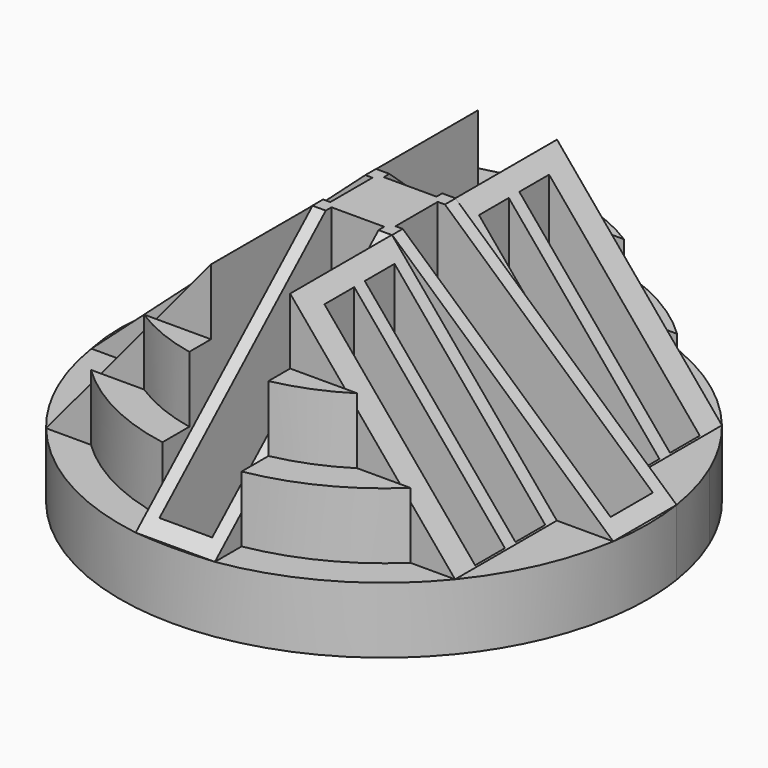
from build123d import *
from build123d import SkipClean  # not in build123d's __all__

# Parameters (mm, degrees)
F2_DEPTH  = 12.7
F3_DEPTH  = 25.4
F4_DEPTH  = 38.1
F5_DEPTH  = 50.8
F6_DEPTH  = 50.8
F7_DEPTH  = 50.8
F11_DEPTH = 15.24
F12_DEPTH = 15.24
F13_DEPTH = 15.24
F15_DEPTH = 15.24
F16_W     = 41.402
F16_H     = 10.16
F16_W_2   = 10.16
F16_H_2   = 41.402
F17_DEPTH = 44.45
F18_DEPTH = 50.8
F21_DEPTH = 24.4856
F19_W     = 29.0068
F19_H     = 7.1628
F22_DEPTH = 44.45
F24_DEPTH = 24.4856
F26_DEPTH = 24.4856
F28_DEPTH = 24.4856


# Not quite as in the source:
# - a feature names something its author has since deleted; it is built from what else it names


with BuildPart() as f2:
    # F1 (on Top) → F2 (new body)
    with BuildSketch(Plane.XY):
        with BuildLine():
            Line((-7.62, 43.7919867099), (-7.62, 50.2252486305))
            ThreePointArc((-7.62, 50.2252486305), (-25.1805025773, 44.1200894146), (-39.3683940318, 32.1056))
            Line((-39.3683940318, 32.1056), (-30.7413882029, 32.1056))
            ThreePointArc((-30.7413882029, 32.1056), (-20.0509833873, 39.670651182), (-7.62, 43.7919867099))
        make_face()
        with BuildLine():
            Line((-30.7413882029, 32.1056), (-39.3683940318, 32.1056))
            ThreePointArc((-39.3683940318, 32.1056), (-43.4950311771, 26.2454236564), (-46.7558464383, 19.8628))
            Line((-46.7558464383, 19.8628), (-39.7652068542, 19.8628))
            ThreePointArc((-39.7652068542, 19.8628), (-35.7808122406, 26.3730160468), (-30.7413882029, 32.1056))
        make_face()
        with BuildLine():
            Line((-39.7652068542, 19.8628), (-46.7558464383, 19.8628))
            ThreePointArc((-46.7558464383, 19.8628), (-48.8754001329, 13.850460709), (-50.2252486305, 7.62))
            Line((-50.2252486305, 7.62), (-43.7919867099, 7.62))
            ThreePointArc((-43.7919867099, 7.62), (-42.2246691762, 13.8881176896), (-39.7652068542, 19.8628))
        make_face()
        with BuildLine():
            Line((-43.7919867099, 7.62), (-50.2252486305, 7.62))
            ThreePointArc((-50.2252486305, 7.62), (-50.8, 0), (-50.2252486305, -7.62))
            Line((-50.2252486305, -7.62), (-43.7919867099, -7.62))
            ThreePointArc((-43.7919867099, -7.62), (-44.45, 0), (-43.7919867099, 7.62))
        make_face()
        with BuildLine():
            ThreePointArc((-50.2252486305, -7.62), (-48.8754001329, -13.850460709), (-46.7558464383, -19.8628))
            Line((-46.7558464383, -19.8628), (-39.7652068542, -19.8628))
            ThreePointArc((-39.7652068542, -19.8628), (-42.2246691762, -13.8881176896), (-43.7919867099, -7.62))
            Line((-43.7919867099, -7.62), (-50.2252486305, -7.62))
        make_face()
        with BuildLine():
            ThreePointArc((-46.7558464383, -19.8628), (-43.4950311771, -26.2454236564), (-39.3683940318, -32.1056))
            Line((-39.3683940318, -32.1056), (-30.7413882029, -32.1056))
            ThreePointArc((-30.7413882029, -32.1056), (-35.7808122406, -26.3730160468), (-39.7652068542, -19.8628))
            Line((-39.7652068542, -19.8628), (-46.7558464383, -19.8628))
        make_face()
        with BuildLine():
            ThreePointArc((-39.3683940318, -32.1056), (-25.1805025773, -44.1200894146), (-7.62, -50.2252486305))
            Line((-7.62, -50.2252486305), (-7.62, -43.7919867099))
            ThreePointArc((-7.62, -43.7919867099), (-20.0509833873, -39.670651182), (-30.7413882029, -32.1056))
            Line((-30.7413882029, -32.1056), (-39.3683940318, -32.1056))
        make_face()
        with BuildLine():
            Line((7.62, 43.7919867099), (7.62, 50.2252486305))
            ThreePointArc((7.62, 50.2252486305), (0, 50.8), (-7.62, 50.2252486305))
            Line((-7.62, 50.2252486305), (-7.62, 43.7919867099))
            ThreePointArc((-7.62, 43.7919867099), (0, 44.45), (7.62, 43.7919867099))
        make_face()
        with BuildLine():
            ThreePointArc((7.62, -50.2252486305), (25.1805025773, -44.1200894146), (39.3683940318, -32.1056))
            Line((39.3683940318, -32.1056), (30.7413882029, -32.1056))
            ThreePointArc((30.7413882029, -32.1056), (20.0509833873, -39.670651182), (7.62, -43.7919867099))
            Line((7.62, -43.7919867099), (7.62, -50.2252486305))
        make_face()
        with BuildLine():
            ThreePointArc((39.3683940318, -32.1056), (43.4950311771, -26.2454236564), (46.7558464383, -19.8628))
            Line((46.7558464383, -19.8628), (39.7652068542, -19.8628))
            ThreePointArc((39.7652068542, -19.8628), (35.7808122406, -26.3730160468), (30.7413882029, -32.1056))
            Line((30.7413882029, -32.1056), (39.3683940318, -32.1056))
        make_face()
        with BuildLine():
            ThreePointArc((46.7558464383, -19.8628), (48.8754001329, -13.850460709), (50.2252486305, -7.62))
            Line((50.2252486305, -7.62), (43.7919867099, -7.62))
            ThreePointArc((43.7919867099, -7.62), (42.2246691762, -13.8881176896), (39.7652068542, -19.8628))
            Line((39.7652068542, -19.8628), (46.7558464383, -19.8628))
        make_face()
        with BuildLine():
            ThreePointArc((50.2252486305, -7.62), (50.6561083702, -3.8208225272), (50.8, 0))
            ThreePointArc((50.8, 0), (50.6561083702, 3.8208225272), (50.2252486305, 7.62))
            Line((50.2252486305, 7.62), (43.7919867099, 7.62))
            ThreePointArc((43.7919867099, 7.62), (44.45, 0), (43.7919867099, -7.62))
            Line((43.7919867099, -7.62), (50.2252486305, -7.62))
        make_face()
        with BuildLine():
            Line((43.7919867099, 7.62), (50.2252486305, 7.62))
            ThreePointArc((50.2252486305, 7.62), (48.8754001329, 13.850460709), (46.7558464383, 19.8628))
            Line((46.7558464383, 19.8628), (39.7652068542, 19.8628))
            ThreePointArc((39.7652068542, 19.8628), (42.2246691762, 13.8881176896), (43.7919867099, 7.62))
        make_face()
        with BuildLine():
            Line((39.7652068542, 19.8628), (46.7558464383, 19.8628))
            ThreePointArc((46.7558464383, 19.8628), (43.4950311771, 26.2454236564), (39.3683940318, 32.1056))
            Line((39.3683940318, 32.1056), (30.7413882029, 32.1056))
            ThreePointArc((30.7413882029, 32.1056), (35.7808122406, 26.3730160468), (39.7652068542, 19.8628))
        make_face()
        with BuildLine():
            Line((30.7413882029, 32.1056), (39.3683940318, 32.1056))
            ThreePointArc((39.3683940318, 32.1056), (25.1805025773, 44.1200894146), (7.62, 50.2252486305))
            Line((7.62, 50.2252486305), (7.62, 43.7919867099))
            ThreePointArc((7.62, 43.7919867099), (20.0509833873, 39.670651182), (30.7413882029, 32.1056))
        make_face()
        with BuildLine():
            ThreePointArc((-7.62, -50.2252486305), (0, -50.8), (7.62, -50.2252486305))
            Line((7.62, -50.2252486305), (7.62, -43.7919867099))
            ThreePointArc((7.62, -43.7919867099), (0, -44.45), (-7.62, -43.7919867099))
            Line((-7.62, -43.7919867099), (-7.62, -50.2252486305))
        make_face()
    extrude(amount=F2_DEPTH)

    # F1 (on Top) → F3 (join)
    with BuildSketch(Plane.XY):
        with BuildLine():
            ThreePointArc((7.62, -43.7919867099), (20.0509833873, -39.670651182), (30.7413882029, -32.1056))
            Line((30.7413882029, -32.1056), (20.5143961315, -32.1056))
            ThreePointArc((20.5143961315, -32.1056), (14.3076984372, -35.3114679025), (7.62, -37.33022368))
            Line((7.62, -37.33022368), (7.62, -43.7919867099))
        make_face()
        with BuildLine():
            ThreePointArc((30.7413882029, -32.1056), (35.7808122406, -26.3730160468), (39.7652068542, -19.8628))
            Line((39.7652068542, -19.8628), (32.5127540538, -19.8628))
            ThreePointArc((32.5127540538, -19.8628), (27.2110492659, -26.667748271), (20.5143961315, -32.1056))
            Line((20.5143961315, -32.1056), (30.7413882029, -32.1056))
        make_face()
        with BuildLine():
            ThreePointArc((39.7652068542, -19.8628), (42.2246691762, -13.8881176896), (43.7919867099, -7.62))
            Line((43.7919867099, -7.62), (37.33022368, -7.62))
            ThreePointArc((37.33022368, -7.62), (35.4539408619, -13.9509167211), (32.5127540538, -19.8628))
            Line((32.5127540538, -19.8628), (39.7652068542, -19.8628))
        make_face()
        with BuildLine():
            ThreePointArc((43.7919867099, -7.62), (44.45, 0), (43.7919867099, 7.62))
            Line((43.7919867099, 7.62), (37.33022368, 7.62))
            ThreePointArc((37.33022368, 7.62), (38.1, 0), (37.33022368, -7.62))
            Line((37.33022368, -7.62), (43.7919867099, -7.62))
        make_face()
        with BuildLine():
            Line((37.33022368, 7.62), (43.7919867099, 7.62))
            ThreePointArc((43.7919867099, 7.62), (42.2246691762, 13.8881176896), (39.7652068542, 19.8628))
            Line((39.7652068542, 19.8628), (32.5127540538, 19.8628))
            ThreePointArc((32.5127540538, 19.8628), (35.4539408619, 13.9509167211), (37.33022368, 7.62))
        make_face()
        with BuildLine():
            Line((32.5127540538, 19.8628), (39.7652068542, 19.8628))
            ThreePointArc((39.7652068542, 19.8628), (35.7808122406, 26.3730160468), (30.7413882029, 32.1056))
            Line((30.7413882029, 32.1056), (20.5143961315, 32.1056))
            ThreePointArc((20.5143961315, 32.1056), (27.2110492659, 26.667748271), (32.5127540538, 19.8628))
        make_face()
        with BuildLine():
            Line((20.5143961315, 32.1056), (30.7413882029, 32.1056))
            ThreePointArc((30.7413882029, 32.1056), (20.0509833873, 39.670651182), (7.62, 43.7919867099))
            Line((7.62, 43.7919867099), (7.62, 37.33022368))
            ThreePointArc((7.62, 37.33022368), (14.3076984372, 35.3114679025), (20.5143961315, 32.1056))
        make_face()
        with BuildLine():
            Line((7.62, 37.33022368), (7.62, 43.7919867099))
            ThreePointArc((7.62, 43.7919867099), (0, 44.45), (-7.62, 43.7919867099))
            Line((-7.62, 43.7919867099), (-7.62, 37.33022368))
            ThreePointArc((-7.62, 37.33022368), (0, 38.1), (7.62, 37.33022368))
        make_face()
        with BuildLine():
            ThreePointArc((-7.62, -43.7919867099), (0, -44.45), (7.62, -43.7919867099))
            Line((7.62, -43.7919867099), (7.62, -37.33022368))
            ThreePointArc((7.62, -37.33022368), (0, -38.1), (-7.62, -37.33022368))
            Line((-7.62, -37.33022368), (-7.62, -43.7919867099))
        make_face()
        with BuildLine():
            Line((-37.33022368, 7.62), (-43.7919867099, 7.62))
            ThreePointArc((-43.7919867099, 7.62), (-44.45, 0), (-43.7919867099, -7.62))
            Line((-43.7919867099, -7.62), (-37.33022368, -7.62))
            ThreePointArc((-37.33022368, -7.62), (-38.1, 0), (-37.33022368, 7.62))
        make_face()
        with BuildLine():
            ThreePointArc((-43.7919867099, -7.62), (-42.2246691762, -13.8881176896), (-39.7652068542, -19.8628))
            Line((-39.7652068542, -19.8628), (-32.5127540538, -19.8628))
            ThreePointArc((-32.5127540538, -19.8628), (-35.4539408619, -13.9509167211), (-37.33022368, -7.62))
            Line((-37.33022368, -7.62), (-43.7919867099, -7.62))
        make_face()
        with BuildLine():
            ThreePointArc((-39.7652068542, -19.8628), (-35.7808122406, -26.3730160468), (-30.7413882029, -32.1056))
            Line((-30.7413882029, -32.1056), (-20.5143961315, -32.1056))
            ThreePointArc((-20.5143961315, -32.1056), (-27.2110492659, -26.667748271), (-32.5127540538, -19.8628))
            Line((-32.5127540538, -19.8628), (-39.7652068542, -19.8628))
        make_face()
        with BuildLine():
            ThreePointArc((-30.7413882029, -32.1056), (-20.0509833873, -39.670651182), (-7.62, -43.7919867099))
            Line((-7.62, -43.7919867099), (-7.62, -37.33022368))
            ThreePointArc((-7.62, -37.33022368), (-14.2009349705, -35.3545392554), (-20.32, -32.2289869527))
            ThreePointArc((-20.32, -32.2289869527), (-20.4172912734, -32.1674403249), (-20.5143961315, -32.1056))
            Line((-20.5143961315, -32.1056), (-30.7413882029, -32.1056))
        make_face()
        with BuildLine():
            Line((-32.5127540538, 19.8628), (-39.7652068542, 19.8628))
            ThreePointArc((-39.7652068542, 19.8628), (-42.2246691762, 13.8881176896), (-43.7919867099, 7.62))
            Line((-43.7919867099, 7.62), (-37.33022368, 7.62))
            ThreePointArc((-37.33022368, 7.62), (-35.4539408619, 13.9509167211), (-32.5127540538, 19.8628))
        make_face()
        with BuildLine():
            Line((-20.5143961315, 32.1056), (-30.7413882029, 32.1056))
            ThreePointArc((-30.7413882029, 32.1056), (-35.7808122406, 26.3730160468), (-39.7652068542, 19.8628))
            Line((-39.7652068542, 19.8628), (-32.5127540538, 19.8628))
            ThreePointArc((-32.5127540538, 19.8628), (-27.2110492659, 26.667748271), (-20.5143961315, 32.1056))
        make_face()
        with BuildLine():
            Line((-7.62, 37.33022368), (-7.62, 43.7919867099))
            ThreePointArc((-7.62, 43.7919867099), (-20.0509833873, 39.670651182), (-30.7413882029, 32.1056))
            Line((-30.7413882029, 32.1056), (-20.5143961315, 32.1056))
            ThreePointArc((-20.5143961315, 32.1056), (-14.3076984372, 35.3114679025), (-7.62, 37.33022368))
        make_face()
    extrude(amount=F3_DEPTH)

    # F1 (on Top) → F4 (join)
    with BuildSketch(Plane.XY):
        with BuildLine():
            ThreePointArc((-7.62, -37.33022368), (0, -38.1), (7.62, -37.33022368))
            Line((7.62, -37.33022368), (7.62, -32.1056))
            Line((7.62, -32.1056), (7.62, -30.8220391928))
            ThreePointArc((7.62, -30.8220391928), (0, -31.75), (-7.62, -30.8220391928))
            Line((-7.62, -30.8220391928), (-7.62, -32.1056))
            Line((-7.62, -32.1056), (-7.62, -37.33022368))
        make_face()
        with BuildLine():
            Line((-7.62, 32.1056), (-7.62, 37.33022368))
            ThreePointArc((-7.62, 37.33022368), (-14.3076984372, 35.3114679025), (-20.5143961315, 32.1056))
            Line((-20.5143961315, 32.1056), (-7.62, 32.1056))
        make_face()
        with BuildLine():
            ThreePointArc((-30.8220391928, 7.62), (-28.4618751136, 14.0706845966), (-24.769571578, 19.8628))
            Line((-24.769571578, 19.8628), (-32.5127540538, 19.8628))
            ThreePointArc((-32.5127540538, 19.8628), (-35.4539408619, 13.9509167211), (-37.33022368, 7.62))
            Line((-37.33022368, 7.62), (-30.8220391928, 7.62))
        make_face()
        with BuildLine():
            Line((-20.32, -32.1056), (-20.5143961315, -32.1056))
            ThreePointArc((-20.5143961315, -32.1056), (-20.4172912734, -32.1674403249), (-20.32, -32.2289869527))
            Line((-20.32, -32.2289869527), (-20.32, -32.1056))
        make_face()
        with BuildLine():
            ThreePointArc((7.62, -37.33022368), (14.3076984372, -35.3114679025), (20.5143961315, -32.1056))
            Line((20.5143961315, -32.1056), (7.62, -32.1056))
            Line((7.62, -32.1056), (7.62, -37.33022368))
        make_face()
        with BuildLine():
            ThreePointArc((32.5127540538, -19.8628), (35.4539408619, -13.9509167211), (37.33022368, -7.62))
            Line((37.33022368, -7.62), (30.8220391928, -7.62))
            ThreePointArc((30.8220391928, -7.62), (28.4618751136, -14.0706845966), (24.769571578, -19.8628))
            Line((24.769571578, -19.8628), (32.5127540538, -19.8628))
        make_face()
        with BuildLine():
            Line((7.62, 32.1056), (20.5143961315, 32.1056))
            ThreePointArc((20.5143961315, 32.1056), (14.3076984372, 35.3114679025), (7.62, 37.33022368))
            Line((7.62, 37.33022368), (7.62, 32.1056))
        make_face()
        with BuildLine():
            Line((7.62, 32.1056), (7.62, 37.33022368))
            ThreePointArc((7.62, 37.33022368), (0, 38.1), (-7.62, 37.33022368))
            Line((-7.62, 37.33022368), (-7.62, 32.1056))
            Line((-7.62, 32.1056), (-7.62, 30.8220391928))
            ThreePointArc((-7.62, 30.8220391928), (0, 31.75), (7.62, 30.8220391928))
            Line((7.62, 30.8220391928), (7.62, 32.1056))
        make_face()
        with BuildLine():
            ThreePointArc((-24.769571578, 19.8628), (-17.0967048776, 26.7537881865), (-7.62, 30.8220391928))
            Line((-7.62, 30.8220391928), (-7.62, 32.1056))
            Line((-7.62, 32.1056), (-20.5143961315, 32.1056))
            ThreePointArc((-20.5143961315, 32.1056), (-27.2110492659, 26.667748271), (-32.5127540538, 19.8628))
            Line((-32.5127540538, 19.8628), (-24.769571578, 19.8628))
        make_face()
        with BuildLine():
            Line((24.769571578, 19.8628), (32.5127540538, 19.8628))
            ThreePointArc((32.5127540538, 19.8628), (27.2110492659, 26.667748271), (20.5143961315, 32.1056))
            Line((20.5143961315, 32.1056), (7.62, 32.1056))
            Line((7.62, 32.1056), (7.62, 30.8220391928))
            ThreePointArc((7.62, 30.8220391928), (17.0967048776, 26.7537881865), (24.769571578, 19.8628))
        make_face()
        with BuildLine():
            ThreePointArc((-30.8220391928, -7.62), (-31.75, 0), (-30.8220391928, 7.62))
            Line((-30.8220391928, 7.62), (-37.33022368, 7.62))
            ThreePointArc((-37.33022368, 7.62), (-38.1, 0), (-37.33022368, -7.62))
            Line((-37.33022368, -7.62), (-30.8220391928, -7.62))
        make_face()
        with BuildLine():
            Line((-32.5127540538, -19.8628), (-24.769571578, -19.8628))
            ThreePointArc((-24.769571578, -19.8628), (-28.4618751136, -14.0706845966), (-30.8220391928, -7.62))
            Line((-30.8220391928, -7.62), (-37.33022368, -7.62))
            ThreePointArc((-37.33022368, -7.62), (-35.4539408619, -13.9509167211), (-32.5127540538, -19.8628))
        make_face()
        with BuildLine():
            Line((-7.62, -32.1056), (-7.62, -30.8220391928))
            ThreePointArc((-7.62, -30.8220391928), (-17.0967048776, -26.7537881865), (-24.769571578, -19.8628))
            Line((-24.769571578, -19.8628), (-32.5127540538, -19.8628))
            ThreePointArc((-32.5127540538, -19.8628), (-27.2110492659, -26.667748271), (-20.5143961315, -32.1056))
            Line((-20.5143961315, -32.1056), (-20.32, -32.1056))
            Line((-20.32, -32.1056), (-7.62, -32.1056))
        make_face()
        with BuildLine():
            ThreePointArc((37.33022368, -7.62), (38.1, 0), (37.33022368, 7.62))
            Line((37.33022368, 7.62), (30.8220391928, 7.62))
            ThreePointArc((30.8220391928, 7.62), (31.5171559977, 3.8381477062), (31.75, 0))
            ThreePointArc((31.75, 0), (31.5171559977, -3.8381477062), (30.8220391928, -7.62))
            Line((30.8220391928, -7.62), (37.33022368, -7.62))
        make_face()
        with BuildLine():
            Line((30.8220391928, 7.62), (37.33022368, 7.62))
            ThreePointArc((37.33022368, 7.62), (35.4539408619, 13.9509167211), (32.5127540538, 19.8628))
            Line((32.5127540538, 19.8628), (24.769571578, 19.8628))
            ThreePointArc((24.769571578, 19.8628), (28.4618751136, 14.0706845966), (30.8220391928, 7.62))
        make_face()
        with BuildLine():
            ThreePointArc((-20.32, -32.2289869527), (-14.2009349705, -35.3545392554), (-7.62, -37.33022368))
            Line((-7.62, -37.33022368), (-7.62, -32.1056))
            Line((-7.62, -32.1056), (-20.32, -32.1056))
            Line((-20.32, -32.1056), (-20.32, -32.2289869527))
        make_face()
        with BuildLine():
            ThreePointArc((20.5143961315, -32.1056), (27.2110492659, -26.667748271), (32.5127540538, -19.8628))
            Line((32.5127540538, -19.8628), (24.769571578, -19.8628))
            ThreePointArc((24.769571578, -19.8628), (17.0967048776, -26.7537881865), (7.62, -30.8220391928))
            Line((7.62, -30.8220391928), (7.62, -32.1056))
            Line((7.62, -32.1056), (20.5143961315, -32.1056))
        make_face()
    extrude(amount=F4_DEPTH)

    # F1 (on Top) → F5 (join)
    with BuildSketch(Plane.XY):
        with BuildLine():
            Line((7.62, 24.230055716), (7.62, 30.8220391928))
            ThreePointArc((7.62, 30.8220391928), (0, 31.75), (-7.62, 30.8220391928))
            Line((-7.62, 30.8220391928), (-7.62, 24.230055716))
            ThreePointArc((-7.62, 24.230055716), (0, 25.4), (7.62, 24.230055716))
        make_face()
        with BuildLine():
            ThreePointArc((-7.62, -30.8220391928), (0, -31.75), (7.62, -30.8220391928))
            Line((7.62, -30.8220391928), (7.62, -24.230055716))
            ThreePointArc((7.62, -24.230055716), (0, -25.4), (-7.62, -24.230055716))
            Line((-7.62, -24.230055716), (-7.62, -30.8220391928))
        make_face()
        with BuildLine():
            ThreePointArc((7.62, -30.8220391928), (17.0967048776, -26.7537881865), (24.769571578, -19.8628))
            Line((24.769571578, -19.8628), (15.8312720954, -19.8628))
            ThreePointArc((15.8312720954, -19.8628), (11.9272281502, -22.4254593856), (7.62, -24.230055716))
            Line((7.62, -24.230055716), (7.62, -30.8220391928))
        make_face()
        with BuildLine():
            Line((15.8312720954, 19.8628), (24.769571578, 19.8628))
            ThreePointArc((24.769571578, 19.8628), (17.0967048776, 26.7537881865), (7.62, 30.8220391928))
            Line((7.62, 30.8220391928), (7.62, 24.230055716))
            ThreePointArc((7.62, 24.230055716), (11.9272281502, 22.4254593856), (15.8312720954, 19.8628))
        make_face()
        with BuildLine():
            Line((-24.230055716, 7.62), (-30.8220391928, 7.62))
            ThreePointArc((-30.8220391928, 7.62), (-31.75, 0), (-30.8220391928, -7.62))
            Line((-30.8220391928, -7.62), (-24.230055716, -7.62))
            ThreePointArc((-24.230055716, -7.62), (-25.4, 0), (-24.230055716, 7.62))
        make_face()
        with BuildLine():
            Line((-7.62, 24.230055716), (-7.62, 30.8220391928))
            ThreePointArc((-7.62, 30.8220391928), (-17.0967048776, 26.7537881865), (-24.769571578, 19.8628))
            Line((-24.769571578, 19.8628), (-15.8312720954, 19.8628))
            ThreePointArc((-15.8312720954, 19.8628), (-11.9272281502, 22.4254593856), (-7.62, 24.230055716))
        make_face()
        with BuildLine():
            ThreePointArc((31.75, 0), (31.5171559977, 3.8381477062), (30.8220391928, 7.62))
            Line((30.8220391928, 7.62), (24.230055716, 7.62))
            ThreePointArc((24.230055716, 7.62), (25.1058102357, 3.8546455618), (25.4, 0))
            ThreePointArc((25.4, 0), (25.1058102357, -3.8546455618), (24.230055716, -7.62))
            Line((24.230055716, -7.62), (30.8220391928, -7.62))
            ThreePointArc((30.8220391928, -7.62), (31.5171559977, -3.8381477062), (31.75, 0))
        make_face()
        with BuildLine():
            ThreePointArc((-30.8220391928, -7.62), (-28.4618751136, -14.0706845966), (-24.769571578, -19.8628))
            Line((-24.769571578, -19.8628), (-20.32, -19.8628))
            Line((-20.32, -19.8628), (-15.8312720954, -19.8628))
            ThreePointArc((-15.8312720954, -19.8628), (-20.9451434577, -14.3687496163), (-24.230055716, -7.62))
            Line((-24.230055716, -7.62), (-30.8220391928, -7.62))
        make_face()
        with BuildLine():
            ThreePointArc((-24.769571578, -19.8628), (-17.0967048776, -26.7537881865), (-7.62, -30.8220391928))
            Line((-7.62, -30.8220391928), (-7.62, -24.230055716))
            ThreePointArc((-7.62, -24.230055716), (-11.9272281502, -22.4254593856), (-15.8312720954, -19.8628))
            Line((-15.8312720954, -19.8628), (-20.32, -19.8628))
            Line((-20.32, -19.8628), (-24.769571578, -19.8628))
        make_face()
    extrude(amount=F5_DEPTH)

    # F1 (on Top) → F6 (join)
    with BuildSketch(Plane.XY):
        with BuildLine():
            ThreePointArc((-7.62, -50.2252486305), (0, -50.8), (7.62, -50.2252486305))
            Line((7.62, -50.2252486305), (7.62, -43.7919867099))
            ThreePointArc((7.62, -43.7919867099), (0, -44.45), (-7.62, -43.7919867099))
            Line((-7.62, -43.7919867099), (-7.62, -50.2252486305))
        make_face()
        with BuildLine():
            ThreePointArc((-7.62, -37.33022368), (0, -38.1), (7.62, -37.33022368))
            Line((7.62, -37.33022368), (7.62, -32.1056))
            Line((7.62, -32.1056), (7.62, -30.8220391928))
            ThreePointArc((7.62, -30.8220391928), (0, -31.75), (-7.62, -30.8220391928))
            Line((-7.62, -30.8220391928), (-7.62, -32.1056))
            Line((-7.62, -32.1056), (-7.62, -37.33022368))
        make_face()
        with BuildLine():
            ThreePointArc((-7.62, -30.8220391928), (0, -31.75), (7.62, -30.8220391928))
            Line((7.62, -30.8220391928), (7.62, -24.230055716))
            ThreePointArc((7.62, -24.230055716), (0, -25.4), (-7.62, -24.230055716))
            Line((-7.62, -24.230055716), (-7.62, -30.8220391928))
        make_face()
        with BuildLine():
            ThreePointArc((-7.62, -43.7919867099), (0, -44.45), (7.62, -43.7919867099))
            Line((7.62, -43.7919867099), (7.62, -37.33022368))
            ThreePointArc((7.62, -37.33022368), (0, -38.1), (-7.62, -37.33022368))
            Line((-7.62, -37.33022368), (-7.62, -43.7919867099))
        make_face()
        with BuildLine():
            Line((7.62, 24.230055716), (7.62, 30.8220391928))
            ThreePointArc((7.62, 30.8220391928), (0, 31.75), (-7.62, 30.8220391928))
            Line((-7.62, 30.8220391928), (-7.62, 24.230055716))
            ThreePointArc((-7.62, 24.230055716), (0, 25.4), (7.62, 24.230055716))
        make_face()
        with BuildLine():
            Line((7.62, 32.1056), (7.62, 37.33022368))
            ThreePointArc((7.62, 37.33022368), (0, 38.1), (-7.62, 37.33022368))
            Line((-7.62, 37.33022368), (-7.62, 32.1056))
            Line((-7.62, 32.1056), (-7.62, 30.8220391928))
            ThreePointArc((-7.62, 30.8220391928), (0, 31.75), (7.62, 30.8220391928))
            Line((7.62, 30.8220391928), (7.62, 32.1056))
        make_face()
        with BuildLine():
            Line((7.62, 37.33022368), (7.62, 43.7919867099))
            ThreePointArc((7.62, 43.7919867099), (0, 44.45), (-7.62, 43.7919867099))
            Line((-7.62, 43.7919867099), (-7.62, 37.33022368))
            ThreePointArc((-7.62, 37.33022368), (0, 38.1), (7.62, 37.33022368))
        make_face()
        with BuildLine():
            Line((7.62, 43.7919867099), (7.62, 50.2252486305))
            ThreePointArc((7.62, 50.2252486305), (0, 50.8), (-7.62, 50.2252486305))
            Line((-7.62, 50.2252486305), (-7.62, 43.7919867099))
            ThreePointArc((-7.62, 43.7919867099), (0, 44.45), (7.62, 43.7919867099))
        make_face()
        Polygon((7.62, -17.78), (7.62, -7.62), (2.54, -7.62), (0, -10.16), align=None)
        Polygon((-2.54, 7.62), (0, 10.16), (-7.62, 17.78), (-7.62, 7.62), align=None)
        Polygon((-7.62, -7.62), (-2.54, -7.62), (-7.62, -2.54), align=None)
        Polygon((-7.62, -17.78), (0, -10.16), (-2.54, -7.62), (-7.62, -7.62), align=None)
        Polygon((7.62, -2.54), (7.62, 2.54), (2.54, 7.62), (0, 7.62), (-2.54, 7.62), (-7.62, 2.54), (-7.62, -2.54), (-2.54, -7.62), (0, -7.62), (2.54, -7.62), align=None)
        Polygon((2.54, 7.62), (7.62, 7.62), (7.62, 17.78), (0, 10.16), align=None)
        with BuildLine():
            ThreePointArc((-7.62, -24.230055716), (0, -25.4), (7.62, -24.230055716))
            Line((7.62, -24.230055716), (7.62, -19.8628))
            Line((7.62, -19.8628), (7.62, -17.78))
            Line((7.62, -17.78), (0, -10.16))
            Line((0, -10.16), (-7.62, -17.78))
            Line((-7.62, -17.78), (-7.62, -19.8628))
            Line((-7.62, -19.8628), (-7.62, -24.230055716))
        make_face()
        with BuildLine():
            Line((7.62, 19.8628), (7.62, 24.230055716))
            ThreePointArc((7.62, 24.230055716), (0, 25.4), (-7.62, 24.230055716))
            Line((-7.62, 24.230055716), (-7.62, 19.8628))
            Line((-7.62, 19.8628), (-7.62, 17.78))
            Line((-7.62, 17.78), (0, 10.16))
            Line((0, 10.16), (7.62, 17.78))
            Line((7.62, 17.78), (7.62, 19.8628))
        make_face()
        Polygon((0, 7.62), (2.54, 7.62), (0, 10.16), (-2.54, 7.62), align=None)
        Polygon((0, -10.16), (2.54, -7.62), (0, -7.62), (-2.54, -7.62), align=None)
        Polygon((-7.62, 2.54), (-2.54, 7.62), (-7.62, 7.62), align=None)
        Polygon((2.54, -7.62), (7.62, -7.62), (7.62, -2.54), align=None)
        Polygon((7.62, 2.54), (7.62, 7.62), (2.54, 7.62), align=None)
    extrude(amount=F6_DEPTH)

    # F1 (on Top) → F7 (join)
    with BuildSketch(Plane.XY):
        with BuildLine():
            Line((-43.7919867099, 7.62), (-50.2252486305, 7.62))
            ThreePointArc((-50.2252486305, 7.62), (-50.8, 0), (-50.2252486305, -7.62))
            Line((-50.2252486305, -7.62), (-43.7919867099, -7.62))
            ThreePointArc((-43.7919867099, -7.62), (-44.45, 0), (-43.7919867099, 7.62))
        make_face()
        with BuildLine():
            Line((-37.33022368, 7.62), (-43.7919867099, 7.62))
            ThreePointArc((-43.7919867099, 7.62), (-44.45, 0), (-43.7919867099, -7.62))
            Line((-43.7919867099, -7.62), (-37.33022368, -7.62))
            ThreePointArc((-37.33022368, -7.62), (-38.1, 0), (-37.33022368, 7.62))
        make_face()
        with BuildLine():
            ThreePointArc((-30.8220391928, -7.62), (-31.75, 0), (-30.8220391928, 7.62))
            Line((-30.8220391928, 7.62), (-37.33022368, 7.62))
            ThreePointArc((-37.33022368, 7.62), (-38.1, 0), (-37.33022368, -7.62))
            Line((-37.33022368, -7.62), (-30.8220391928, -7.62))
        make_face()
        with BuildLine():
            Line((-24.230055716, 7.62), (-30.8220391928, 7.62))
            ThreePointArc((-30.8220391928, 7.62), (-31.75, 0), (-30.8220391928, -7.62))
            Line((-30.8220391928, -7.62), (-24.230055716, -7.62))
            ThreePointArc((-24.230055716, -7.62), (-25.4, 0), (-24.230055716, 7.62))
        make_face()
        with BuildLine():
            Line((-17.78, 7.62), (-24.230055716, 7.62))
            ThreePointArc((-24.230055716, 7.62), (-25.4, 0), (-24.230055716, -7.62))
            Line((-24.230055716, -7.62), (-17.78, -7.62))
            Line((-17.78, -7.62), (-10.16, 0))
            Line((-10.16, 0), (-17.78, 7.62))
        make_face()
        Polygon((-7.62, -7.62), (-2.54, -7.62), (-7.62, -2.54), align=None)
        with BuildLine():
            ThreePointArc((25.4, 0), (25.1058102357, 3.8546455618), (24.230055716, 7.62))
            Line((24.230055716, 7.62), (17.78, 7.62))
            Line((17.78, 7.62), (10.16, 0))
            Line((10.16, 0), (17.78, -7.62))
            Line((17.78, -7.62), (24.230055716, -7.62))
            ThreePointArc((24.230055716, -7.62), (25.1058102357, -3.8546455618), (25.4, 0))
        make_face()
        with BuildLine():
            ThreePointArc((31.75, 0), (31.5171559977, 3.8381477062), (30.8220391928, 7.62))
            Line((30.8220391928, 7.62), (24.230055716, 7.62))
            ThreePointArc((24.230055716, 7.62), (25.1058102357, 3.8546455618), (25.4, 0))
            ThreePointArc((25.4, 0), (25.1058102357, -3.8546455618), (24.230055716, -7.62))
            Line((24.230055716, -7.62), (30.8220391928, -7.62))
            ThreePointArc((30.8220391928, -7.62), (31.5171559977, -3.8381477062), (31.75, 0))
        make_face()
        with BuildLine():
            ThreePointArc((37.33022368, -7.62), (38.1, 0), (37.33022368, 7.62))
            Line((37.33022368, 7.62), (30.8220391928, 7.62))
            ThreePointArc((30.8220391928, 7.62), (31.5171559977, 3.8381477062), (31.75, 0))
            ThreePointArc((31.75, 0), (31.5171559977, -3.8381477062), (30.8220391928, -7.62))
            Line((30.8220391928, -7.62), (37.33022368, -7.62))
        make_face()
        with BuildLine():
            ThreePointArc((43.7919867099, -7.62), (44.45, 0), (43.7919867099, 7.62))
            Line((43.7919867099, 7.62), (37.33022368, 7.62))
            ThreePointArc((37.33022368, 7.62), (38.1, 0), (37.33022368, -7.62))
            Line((37.33022368, -7.62), (43.7919867099, -7.62))
        make_face()
        with BuildLine():
            ThreePointArc((50.2252486305, -7.62), (50.6561083702, -3.8208225272), (50.8, 0))
            ThreePointArc((50.8, 0), (50.6561083702, 3.8208225272), (50.2252486305, 7.62))
            Line((50.2252486305, 7.62), (43.7919867099, 7.62))
            ThreePointArc((43.7919867099, 7.62), (44.45, 0), (43.7919867099, -7.62))
            Line((43.7919867099, -7.62), (50.2252486305, -7.62))
        make_face()
        Polygon((-10.16, 0), (-17.78, -7.62), (-7.62, -7.62), (-7.62, -2.54), align=None)
        Polygon((10.16, 0), (17.78, 7.62), (7.62, 7.62), (7.62, 2.54), align=None)
        Polygon((-7.62, -2.54), (-7.62, 2.54), (-10.16, 0), align=None)
        Polygon((7.62, -2.54), (10.16, 0), (7.62, 2.54), align=None)
        Polygon((-7.62, 7.62), (-17.78, 7.62), (-10.16, 0), (-7.62, 2.54), align=None)
        Polygon((7.62, -7.62), (17.78, -7.62), (10.16, 0), (7.62, -2.54), align=None)
        with BuildLine():
            ThreePointArc((-15.8312720954, -19.8628), (-11.9272281502, -22.4254593856), (-7.62, -24.230055716))
            Line((-7.62, -24.230055716), (-7.62, -19.8628))
            Line((-7.62, -19.8628), (-15.8312720954, -19.8628))
        make_face()
        with BuildLine():
            ThreePointArc((-24.230055716, -7.62), (-20.9451434577, -14.3687496163), (-15.8312720954, -19.8628))
            Line((-15.8312720954, -19.8628), (-7.62, -19.8628))
            Line((-7.62, -19.8628), (-7.62, -17.78))
            Line((-7.62, -17.78), (-7.62, -7.62))
            Line((-7.62, -7.62), (-17.78, -7.62))
            Line((-17.78, -7.62), (-24.230055716, -7.62))
        make_face()
        with BuildLine():
            ThreePointArc((15.8312720954, -19.8628), (20.9451434577, -14.3687496163), (24.230055716, -7.62))
            Line((24.230055716, -7.62), (17.78, -7.62))
            Line((17.78, -7.62), (7.62, -7.62))
            Line((7.62, -7.62), (7.62, -17.78))
            Line((7.62, -17.78), (7.62, -19.8628))
            Line((7.62, -19.8628), (15.8312720954, -19.8628))
        make_face()
        with BuildLine():
            Line((17.78, 7.62), (24.230055716, 7.62))
            ThreePointArc((24.230055716, 7.62), (20.9451434577, 14.3687496163), (15.8312720954, 19.8628))
            Line((15.8312720954, 19.8628), (7.62, 19.8628))
            Line((7.62, 19.8628), (7.62, 17.78))
            Line((7.62, 17.78), (7.62, 7.62))
            Line((7.62, 7.62), (17.78, 7.62))
        make_face()
        with BuildLine():
            Line((-7.62, 19.8628), (-15.8312720954, 19.8628))
            ThreePointArc((-15.8312720954, 19.8628), (-20.9451434577, 14.3687496163), (-24.230055716, 7.62))
            Line((-24.230055716, 7.62), (-17.78, 7.62))
            Line((-17.78, 7.62), (-7.62, 7.62))
            Line((-7.62, 7.62), (-7.62, 17.78))
            Line((-7.62, 17.78), (-7.62, 19.8628))
        make_face()
    extrude(amount=F7_DEPTH)

    # F8 (on face) → F11 (cut)
    with BuildSketch(Plane.XZ.offset(7.62)):
        Polygon((-54.3301515281, 14.2320003361), (-50.2252486305, 12.7), (-7.6606776565, 50.8), (-7.6606776565, 64.8320242763), (-55.9246055782, 64.8320242763), align=None)
    extrude(amount=-F11_DEPTH, mode=Mode.SUBTRACT)

    # F9 (on face) → F12 (cut)
    with BuildSketch(Plane.XZ.offset(7.62)):
        Polygon((7.6703908853, 50.8), (50.2252486305, 12.7), (55.3924329579, 12.7), (55.3924329579, 55.8396019042), (7.6703908853, 53.9275594056), align=None)
    extrude(amount=-F12_DEPTH, mode=Mode.SUBTRACT)

    # F10 (on face) → F13 (cut)
    with BuildSketch(Plane.YZ.offset(7.62)):
        Polygon((-56.448481977, 14.0103092417), (-50.2252486305, 12.7), (-7.6625170186, 50.8), (-7.6625170186, 52.6358112693), (-57.5197674334, 52.6358112693), align=None)
    extrude(amount=-F13_DEPTH, mode=Mode.SUBTRACT)

    # F14 (on face) → F15 (cut)
    with BuildSketch(Plane(origin=(-7.62, 0, 0), x_dir=(0, -1, 0), z_dir=(-1, 0, 0))):
        Polygon((-54.0386848152, 12.7), (-50.2252486305, 12.7), (-7.6549332589, 50.8), (-7.6549332589, 52.5853484869), (-58.2393705845, 53.2422102988), align=None)
    extrude(amount=-F15_DEPTH, mode=Mode.SUBTRACT)

    # F16 (on offset) → F17 (cut)
    with BuildSketch(Plane.XY.offset(50.8)):
        with Locations((26.9842486305, 0)):
            Rectangle(F16_W, F16_H)
        with Locations((-26.9842486305, 0)):
            Rectangle(F16_W, F16_H)
        with Locations((0, 26.9842486305)):
            Rectangle(F16_W_2, F16_H_2)
        with Locations((0, -26.9842486305)):
            Rectangle(F16_W_2, F16_H_2)
    extrude(amount=-F17_DEPTH, mode=Mode.SUBTRACT)

    # F1 (on Top) → F18 (join)
    with BuildSketch(Plane.XY):
        with BuildLine():
            ThreePointArc((-24.230055716, -7.62), (-20.9451434577, -14.3687496163), (-15.8312720954, -19.8628))
            Line((-15.8312720954, -19.8628), (-7.62, -19.8628))
            Line((-7.62, -19.8628), (-7.62, -17.78))
            Line((-7.62, -17.78), (-7.62, -7.62))
            Line((-7.62, -7.62), (-17.78, -7.62))
            Line((-17.78, -7.62), (-24.230055716, -7.62))
        make_face()
        with BuildLine():
            ThreePointArc((-30.8220391928, -7.62), (-28.4618751136, -14.0706845966), (-24.769571578, -19.8628))
            Line((-24.769571578, -19.8628), (-20.32, -19.8628))
            Line((-20.32, -19.8628), (-15.8312720954, -19.8628))
            ThreePointArc((-15.8312720954, -19.8628), (-20.9451434577, -14.3687496163), (-24.230055716, -7.62))
            Line((-24.230055716, -7.62), (-30.8220391928, -7.62))
        make_face()
        with BuildLine():
            Line((-32.5127540538, -19.8628), (-24.769571578, -19.8628))
            ThreePointArc((-24.769571578, -19.8628), (-28.4618751136, -14.0706845966), (-30.8220391928, -7.62))
            Line((-30.8220391928, -7.62), (-37.33022368, -7.62))
            ThreePointArc((-37.33022368, -7.62), (-35.4539408619, -13.9509167211), (-32.5127540538, -19.8628))
        make_face()
        with BuildLine():
            ThreePointArc((-43.7919867099, -7.62), (-42.2246691762, -13.8881176896), (-39.7652068542, -19.8628))
            Line((-39.7652068542, -19.8628), (-32.5127540538, -19.8628))
            ThreePointArc((-32.5127540538, -19.8628), (-35.4539408619, -13.9509167211), (-37.33022368, -7.62))
            Line((-37.33022368, -7.62), (-43.7919867099, -7.62))
        make_face()
        with BuildLine():
            ThreePointArc((-50.2252486305, -7.62), (-48.8754001329, -13.850460709), (-46.7558464383, -19.8628))
            Line((-46.7558464383, -19.8628), (-39.7652068542, -19.8628))
            ThreePointArc((-39.7652068542, -19.8628), (-42.2246691762, -13.8881176896), (-43.7919867099, -7.62))
            Line((-43.7919867099, -7.62), (-50.2252486305, -7.62))
        make_face()
        with BuildLine():
            ThreePointArc((-15.8312720954, -19.8628), (-11.9272281502, -22.4254593856), (-7.62, -24.230055716))
            Line((-7.62, -24.230055716), (-7.62, -19.8628))
            Line((-7.62, -19.8628), (-15.8312720954, -19.8628))
        make_face()
        with BuildLine():
            ThreePointArc((-24.769571578, -19.8628), (-17.0967048776, -26.7537881865), (-7.62, -30.8220391928))
            Line((-7.62, -30.8220391928), (-7.62, -24.230055716))
            ThreePointArc((-7.62, -24.230055716), (-11.9272281502, -22.4254593856), (-15.8312720954, -19.8628))
            Line((-15.8312720954, -19.8628), (-20.32, -19.8628))
            Line((-20.32, -19.8628), (-24.769571578, -19.8628))
        make_face()
        with BuildLine():
            Line((-7.62, -32.1056), (-7.62, -30.8220391928))
            ThreePointArc((-7.62, -30.8220391928), (-17.0967048776, -26.7537881865), (-24.769571578, -19.8628))
            Line((-24.769571578, -19.8628), (-32.5127540538, -19.8628))
            ThreePointArc((-32.5127540538, -19.8628), (-27.2110492659, -26.667748271), (-20.5143961315, -32.1056))
            Line((-20.5143961315, -32.1056), (-20.32, -32.1056))
            Line((-20.32, -32.1056), (-7.62, -32.1056))
        make_face()
        with BuildLine():
            ThreePointArc((-39.7652068542, -19.8628), (-35.7808122406, -26.3730160468), (-30.7413882029, -32.1056))
            Line((-30.7413882029, -32.1056), (-20.5143961315, -32.1056))
            ThreePointArc((-20.5143961315, -32.1056), (-27.2110492659, -26.667748271), (-32.5127540538, -19.8628))
            Line((-32.5127540538, -19.8628), (-39.7652068542, -19.8628))
        make_face()
        with BuildLine():
            ThreePointArc((-46.7558464383, -19.8628), (-43.4950311771, -26.2454236564), (-39.3683940318, -32.1056))
            Line((-39.3683940318, -32.1056), (-30.7413882029, -32.1056))
            ThreePointArc((-30.7413882029, -32.1056), (-35.7808122406, -26.3730160468), (-39.7652068542, -19.8628))
            Line((-39.7652068542, -19.8628), (-46.7558464383, -19.8628))
        make_face()
        with BuildLine():
            Line((-30.7413882029, 32.1056), (-39.3683940318, 32.1056))
            ThreePointArc((-39.3683940318, 32.1056), (-43.4950311771, 26.2454236564), (-46.7558464383, 19.8628))
            Line((-46.7558464383, 19.8628), (-39.7652068542, 19.8628))
            ThreePointArc((-39.7652068542, 19.8628), (-35.7808122406, 26.3730160468), (-30.7413882029, 32.1056))
        make_face()
        with BuildLine():
            Line((-39.7652068542, 19.8628), (-46.7558464383, 19.8628))
            ThreePointArc((-46.7558464383, 19.8628), (-48.8754001329, 13.850460709), (-50.2252486305, 7.62))
            Line((-50.2252486305, 7.62), (-43.7919867099, 7.62))
            ThreePointArc((-43.7919867099, 7.62), (-42.2246691762, 13.8881176896), (-39.7652068542, 19.8628))
        make_face()
        with BuildLine():
            Line((-20.5143961315, 32.1056), (-30.7413882029, 32.1056))
            ThreePointArc((-30.7413882029, 32.1056), (-35.7808122406, 26.3730160468), (-39.7652068542, 19.8628))
            Line((-39.7652068542, 19.8628), (-32.5127540538, 19.8628))
            ThreePointArc((-32.5127540538, 19.8628), (-27.2110492659, 26.667748271), (-20.5143961315, 32.1056))
        make_face()
        with BuildLine():
            Line((-32.5127540538, 19.8628), (-39.7652068542, 19.8628))
            ThreePointArc((-39.7652068542, 19.8628), (-42.2246691762, 13.8881176896), (-43.7919867099, 7.62))
            Line((-43.7919867099, 7.62), (-37.33022368, 7.62))
            ThreePointArc((-37.33022368, 7.62), (-35.4539408619, 13.9509167211), (-32.5127540538, 19.8628))
        make_face()
        with BuildLine():
            ThreePointArc((-24.769571578, 19.8628), (-17.0967048776, 26.7537881865), (-7.62, 30.8220391928))
            Line((-7.62, 30.8220391928), (-7.62, 32.1056))
            Line((-7.62, 32.1056), (-20.5143961315, 32.1056))
            ThreePointArc((-20.5143961315, 32.1056), (-27.2110492659, 26.667748271), (-32.5127540538, 19.8628))
            Line((-32.5127540538, 19.8628), (-24.769571578, 19.8628))
        make_face()
        with BuildLine():
            ThreePointArc((-30.8220391928, 7.62), (-28.4618751136, 14.0706845966), (-24.769571578, 19.8628))
            Line((-24.769571578, 19.8628), (-32.5127540538, 19.8628))
            ThreePointArc((-32.5127540538, 19.8628), (-35.4539408619, 13.9509167211), (-37.33022368, 7.62))
            Line((-37.33022368, 7.62), (-30.8220391928, 7.62))
        make_face()
        with BuildLine():
            Line((-7.62, 24.230055716), (-7.62, 30.8220391928))
            ThreePointArc((-7.62, 30.8220391928), (-17.0967048776, 26.7537881865), (-24.769571578, 19.8628))
            Line((-24.769571578, 19.8628), (-15.8312720954, 19.8628))
            ThreePointArc((-15.8312720954, 19.8628), (-11.9272281502, 22.4254593856), (-7.62, 24.230055716))
        make_face()
        with BuildLine():
            Line((-15.8312720954, 19.8628), (-24.769571578, 19.8628))
            ThreePointArc((-24.769571578, 19.8628), (-28.4618751136, 14.0706845966), (-30.8220391928, 7.62))
            Line((-30.8220391928, 7.62), (-24.230055716, 7.62))
            ThreePointArc((-24.230055716, 7.62), (-20.9451434577, 14.3687496163), (-15.8312720954, 19.8628))
        make_face()
        with BuildLine():
            Line((-7.62, 19.8628), (-15.8312720954, 19.8628))
            ThreePointArc((-15.8312720954, 19.8628), (-20.9451434577, 14.3687496163), (-24.230055716, 7.62))
            Line((-24.230055716, 7.62), (-17.78, 7.62))
            Line((-17.78, 7.62), (-7.62, 7.62))
            Line((-7.62, 7.62), (-7.62, 17.78))
            Line((-7.62, 17.78), (-7.62, 19.8628))
        make_face()
        with BuildLine():
            Line((-7.62, 19.8628), (-7.62, 24.230055716))
            ThreePointArc((-7.62, 24.230055716), (-11.9272281502, 22.4254593856), (-15.8312720954, 19.8628))
            Line((-15.8312720954, 19.8628), (-7.62, 19.8628))
        make_face()
        with BuildLine():
            ThreePointArc((7.62, -24.230055716), (11.9272281502, -22.4254593856), (15.8312720954, -19.8628))
            Line((15.8312720954, -19.8628), (7.62, -19.8628))
            Line((7.62, -19.8628), (7.62, -24.230055716))
        make_face()
        with BuildLine():
            ThreePointArc((7.62, -30.8220391928), (17.0967048776, -26.7537881865), (24.769571578, -19.8628))
            Line((24.769571578, -19.8628), (15.8312720954, -19.8628))
            ThreePointArc((15.8312720954, -19.8628), (11.9272281502, -22.4254593856), (7.62, -24.230055716))
            Line((7.62, -24.230055716), (7.62, -30.8220391928))
        make_face()
        with BuildLine():
            ThreePointArc((30.7413882029, -32.1056), (35.7808122406, -26.3730160468), (39.7652068542, -19.8628))
            Line((39.7652068542, -19.8628), (32.5127540538, -19.8628))
            ThreePointArc((32.5127540538, -19.8628), (27.2110492659, -26.667748271), (20.5143961315, -32.1056))
            Line((20.5143961315, -32.1056), (30.7413882029, -32.1056))
        make_face()
        with BuildLine():
            ThreePointArc((20.5143961315, -32.1056), (27.2110492659, -26.667748271), (32.5127540538, -19.8628))
            Line((32.5127540538, -19.8628), (24.769571578, -19.8628))
            ThreePointArc((24.769571578, -19.8628), (17.0967048776, -26.7537881865), (7.62, -30.8220391928))
            Line((7.62, -30.8220391928), (7.62, -32.1056))
            Line((7.62, -32.1056), (20.5143961315, -32.1056))
        make_face()
        with BuildLine():
            ThreePointArc((39.3683940318, -32.1056), (43.4950311771, -26.2454236564), (46.7558464383, -19.8628))
            Line((46.7558464383, -19.8628), (39.7652068542, -19.8628))
            ThreePointArc((39.7652068542, -19.8628), (35.7808122406, -26.3730160468), (30.7413882029, -32.1056))
            Line((30.7413882029, -32.1056), (39.3683940318, -32.1056))
        make_face()
        with BuildLine():
            ThreePointArc((15.8312720954, -19.8628), (20.9451434577, -14.3687496163), (24.230055716, -7.62))
            Line((24.230055716, -7.62), (17.78, -7.62))
            Line((17.78, -7.62), (7.62, -7.62))
            Line((7.62, -7.62), (7.62, -17.78))
            Line((7.62, -17.78), (7.62, -19.8628))
            Line((7.62, -19.8628), (15.8312720954, -19.8628))
        make_face()
        with BuildLine():
            ThreePointArc((24.769571578, -19.8628), (28.4618751136, -14.0706845966), (30.8220391928, -7.62))
            Line((30.8220391928, -7.62), (24.230055716, -7.62))
            ThreePointArc((24.230055716, -7.62), (20.9451434577, -14.3687496163), (15.8312720954, -19.8628))
            Line((15.8312720954, -19.8628), (24.769571578, -19.8628))
        make_face()
        with BuildLine():
            ThreePointArc((32.5127540538, -19.8628), (35.4539408619, -13.9509167211), (37.33022368, -7.62))
            Line((37.33022368, -7.62), (30.8220391928, -7.62))
            ThreePointArc((30.8220391928, -7.62), (28.4618751136, -14.0706845966), (24.769571578, -19.8628))
            Line((24.769571578, -19.8628), (32.5127540538, -19.8628))
        make_face()
        with BuildLine():
            ThreePointArc((39.7652068542, -19.8628), (42.2246691762, -13.8881176896), (43.7919867099, -7.62))
            Line((43.7919867099, -7.62), (37.33022368, -7.62))
            ThreePointArc((37.33022368, -7.62), (35.4539408619, -13.9509167211), (32.5127540538, -19.8628))
            Line((32.5127540538, -19.8628), (39.7652068542, -19.8628))
        make_face()
        with BuildLine():
            ThreePointArc((46.7558464383, -19.8628), (48.8754001329, -13.850460709), (50.2252486305, -7.62))
            Line((50.2252486305, -7.62), (43.7919867099, -7.62))
            ThreePointArc((43.7919867099, -7.62), (42.2246691762, -13.8881176896), (39.7652068542, -19.8628))
            Line((39.7652068542, -19.8628), (46.7558464383, -19.8628))
        make_face()
        with BuildLine():
            Line((17.78, 7.62), (24.230055716, 7.62))
            ThreePointArc((24.230055716, 7.62), (20.9451434577, 14.3687496163), (15.8312720954, 19.8628))
            Line((15.8312720954, 19.8628), (7.62, 19.8628))
            Line((7.62, 19.8628), (7.62, 17.78))
            Line((7.62, 17.78), (7.62, 7.62))
            Line((7.62, 7.62), (17.78, 7.62))
        make_face()
        with BuildLine():
            Line((24.230055716, 7.62), (30.8220391928, 7.62))
            ThreePointArc((30.8220391928, 7.62), (28.4618751136, 14.0706845966), (24.769571578, 19.8628))
            Line((24.769571578, 19.8628), (15.8312720954, 19.8628))
            ThreePointArc((15.8312720954, 19.8628), (20.9451434577, 14.3687496163), (24.230055716, 7.62))
        make_face()
        with BuildLine():
            Line((30.8220391928, 7.62), (37.33022368, 7.62))
            ThreePointArc((37.33022368, 7.62), (35.4539408619, 13.9509167211), (32.5127540538, 19.8628))
            Line((32.5127540538, 19.8628), (24.769571578, 19.8628))
            ThreePointArc((24.769571578, 19.8628), (28.4618751136, 14.0706845966), (30.8220391928, 7.62))
        make_face()
        with BuildLine():
            Line((37.33022368, 7.62), (43.7919867099, 7.62))
            ThreePointArc((43.7919867099, 7.62), (42.2246691762, 13.8881176896), (39.7652068542, 19.8628))
            Line((39.7652068542, 19.8628), (32.5127540538, 19.8628))
            ThreePointArc((32.5127540538, 19.8628), (35.4539408619, 13.9509167211), (37.33022368, 7.62))
        make_face()
        with BuildLine():
            Line((43.7919867099, 7.62), (50.2252486305, 7.62))
            ThreePointArc((50.2252486305, 7.62), (48.8754001329, 13.850460709), (46.7558464383, 19.8628))
            Line((46.7558464383, 19.8628), (39.7652068542, 19.8628))
            ThreePointArc((39.7652068542, 19.8628), (42.2246691762, 13.8881176896), (43.7919867099, 7.62))
        make_face()
        with BuildLine():
            Line((39.7652068542, 19.8628), (46.7558464383, 19.8628))
            ThreePointArc((46.7558464383, 19.8628), (43.4950311771, 26.2454236564), (39.3683940318, 32.1056))
            Line((39.3683940318, 32.1056), (30.7413882029, 32.1056))
            ThreePointArc((30.7413882029, 32.1056), (35.7808122406, 26.3730160468), (39.7652068542, 19.8628))
        make_face()
        with BuildLine():
            Line((32.5127540538, 19.8628), (39.7652068542, 19.8628))
            ThreePointArc((39.7652068542, 19.8628), (35.7808122406, 26.3730160468), (30.7413882029, 32.1056))
            Line((30.7413882029, 32.1056), (20.5143961315, 32.1056))
            ThreePointArc((20.5143961315, 32.1056), (27.2110492659, 26.667748271), (32.5127540538, 19.8628))
        make_face()
        with BuildLine():
            Line((24.769571578, 19.8628), (32.5127540538, 19.8628))
            ThreePointArc((32.5127540538, 19.8628), (27.2110492659, 26.667748271), (20.5143961315, 32.1056))
            Line((20.5143961315, 32.1056), (7.62, 32.1056))
            Line((7.62, 32.1056), (7.62, 30.8220391928))
            ThreePointArc((7.62, 30.8220391928), (17.0967048776, 26.7537881865), (24.769571578, 19.8628))
        make_face()
        with BuildLine():
            Line((15.8312720954, 19.8628), (24.769571578, 19.8628))
            ThreePointArc((24.769571578, 19.8628), (17.0967048776, 26.7537881865), (7.62, 30.8220391928))
            Line((7.62, 30.8220391928), (7.62, 24.230055716))
            ThreePointArc((7.62, 24.230055716), (11.9272281502, 22.4254593856), (15.8312720954, 19.8628))
        make_face()
        with BuildLine():
            Line((7.62, 19.8628), (15.8312720954, 19.8628))
            ThreePointArc((15.8312720954, 19.8628), (11.9272281502, 22.4254593856), (7.62, 24.230055716))
            Line((7.62, 24.230055716), (7.62, 19.8628))
        make_face()
    with SkipClean():  # cleaning this boolean's faces spoils the solid; the shape is the same uncleaned
        extrude(amount=F18_DEPTH)

    # F20 (on face) → F21 (cut)
    with BuildSketch(Plane.XZ.offset(32.1056)):
        Polygon((-39.3683940318, 12.7), (-7.62, 50.8), (-7.62, 65.6115189195), (-60.1087734103, 65.6115189195), (-60.1087734103, 12.7), align=None)
    with SkipClean():  # cleaning this boolean's faces spoils the solid; the shape is the same uncleaned
        extrude(amount=-F21_DEPTH, mode=Mode.SUBTRACT)

    # F19 (on offset) → F22 (cut)
    with BuildSketch(Plane.XY.offset(50.8)):
        with Locations((-24.6634, -13.7414)):
            Rectangle(F19_W, F19_H)
        with Locations((-24.6634, -23.4442)):
            Rectangle(F19_W, F19_H)
        with Locations((-24.6634, 13.7414)):
            Rectangle(F19_W, F19_H)
        with Locations((-24.6634, 23.4442)):
            Rectangle(F19_W, F19_H)
        with Locations((24.6634, 23.4442)):
            Rectangle(F19_W, F19_H)
        with Locations((24.6634, 13.7414)):
            Rectangle(F19_W, F19_H)
        with Locations((24.6634, -13.7414)):
            Rectangle(F19_W, F19_H)
        with Locations((24.6634, -23.4442)):
            Rectangle(F19_W, F19_H)
    with SkipClean():  # cleaning this boolean's faces spoils the solid; the shape is the same uncleaned
        extrude(amount=-F22_DEPTH, mode=Mode.SUBTRACT)

    # F23 (on face) → F24 (cut)
    with BuildSketch(Plane(origin=(0, 32.1056, 0), x_dir=(-1, 0, 0), z_dir=(0, 1, 0))):
        Polygon((7.62, 58.9498654008), (7.62, 50.8), (39.3683940318, 12.7), (63.3994191885, 12.7), (63.3994191885, 58.9498654008), align=None)
    extrude(amount=-F24_DEPTH, mode=Mode.SUBTRACT)

    # F25 (on face) → F26 (cut)
    with BuildSketch(Plane(origin=(0, 32.1056, 0), x_dir=(-1, 0, 0), z_dir=(0, 1, 0))):
        Polygon((-39.3683940318, 12.7), (-7.62, 50.8), (-7.62, 60.825034976), (-64.4157677889, 60.825034976), (-64.4157677889, 12.7), align=None)
    extrude(amount=-F26_DEPTH, mode=Mode.SUBTRACT)

    # F27 (on face) → F28 (cut)
    with BuildSketch(Plane.XZ.offset(32.1056)):
        Polygon((7.62, 58.3216398954), (7.62, 50.8), (39.3683940318, 12.7), (79.0987238288, 12.7), (79.0987238288, 63.607044518), align=None)
    extrude(amount=-F28_DEPTH, mode=Mode.SUBTRACT)


solid = f2.part
